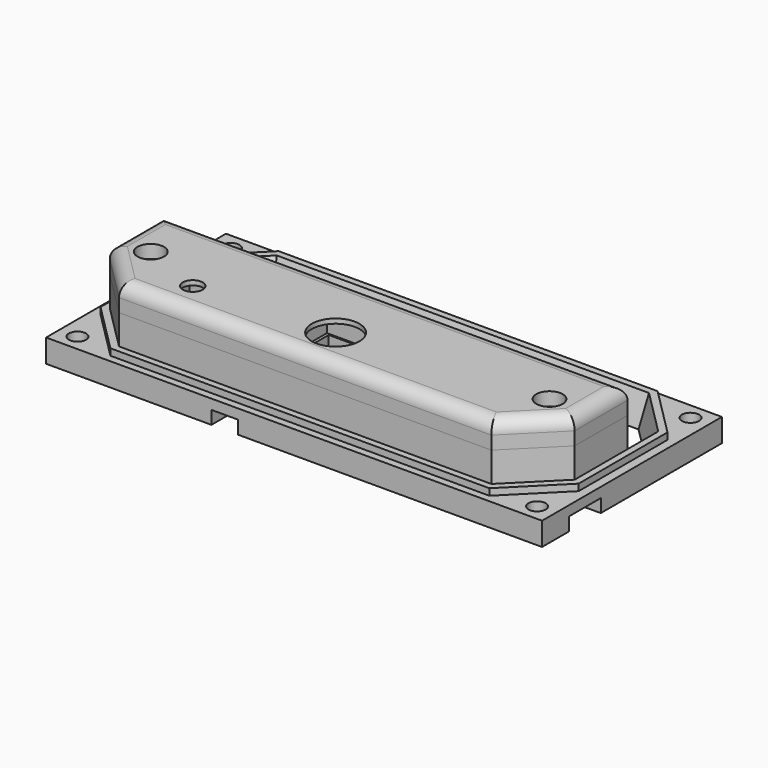
from build123d import *

# Parameters (mm, degrees)
F0_W              = 75
F0_H              = 34
F0_R              = 1.3
F1_DEPTH          = 3.5
F3_DEPTH          = 1
F5_DEPTH          = 5
F11_DEPTH         = 9
F12_W             = 15
F12_H             = 10
F13_DEPTH         = 8.5
F14_W             = 7.3
F14_H             = 4.5
F15_DEPTH         = 5
F16_W             = 9
F16_H             = 10
F16_W_2           = 7
F16_H_2           = 4
F17_DEPTH         = 25
F18_W             = 2
F18_H             = 5
F19_DEPTH         = 10
F20_W             = 6
F20_H             = 2
F21_DEPTH         = 25
F22_R             = 0.8
F23_DEPTH         = 5
F26_DEPTH         = 4
F27_R             = 3.6
F27_R_2           = 1.5
F28_DEPTH         = 25
F29_W             = 13
F29_H             = 10.5
F29_W_2           = 8
F29_H_2           = 5
F30_DEPTH         = 3.3
F31_W             = 2
F31_H             = 4
F32_DEPTH         = 7
F33_W             = 4
F33_H             = 2
F34_DEPTH         = 25
F36_D             = 2
F36_DEPTH         = 10
F36_CBORE_D       = 4
F36_CBORE_DEPTH   = 2
F36_TIP           = 0.600860619
F36_2_D           = 2
F36_2_DEPTH       = 10
F36_2_CBORE_D     = 4
F36_2_CBORE_DEPTH = 2
F36_2_TIP         = 0.600860619
F37_R             = 2


with BuildPart() as f1:
    # F0 (on Top) → F1 (new body)
    with BuildSketch(Plane.XY):
        Rectangle(F0_W, F0_H)
        with Locations((-34.75, -14.5)):
            Circle(F0_R, mode=Mode.SUBTRACT)
        with Locations((34.75, -14.5)):
            Circle(F0_R, mode=Mode.SUBTRACT)
        with Locations((-34.75, 14.5)):
            Circle(F0_R, mode=Mode.SUBTRACT)
        with Locations((34.75, 14.5)):
            Circle(F0_R, mode=Mode.SUBTRACT)
    extrude(amount=F1_DEPTH)

    # F2 (on face) → F3 (join)
    with BuildSketch(Plane.XY.offset(3.5)):
        Polygon((28.65, 15.9), (-28.65, 15.9), (-36.15, 8.4), (-36.15, -8.4), (-28.65, -15.9), (28.65, -15.9), (36.15, -8.4), (36.15, 8.4), align=None)
    extrude(amount=F3_DEPTH)

    # F4 (on face) → F5 (cut)
    with BuildSketch(Plane.XY.offset(4.5)):
        Polygon((28.15, 14.9), (-28.15, 14.9), (-35.15, 7.9), (-35.15, -7.9), (-28.15, -14.9), (28.15, -14.9), (35.15, -7.9), (35.15, 7.9), align=None)
    extrude(amount=-F5_DEPTH, mode=Mode.SUBTRACT)

    # F9: sweep along a path in F8
    with BuildLine(Plane.XY.offset(4.5)) as f9_path:
        Line((-35.15, 2.1), (-35.15, 7.9))
        Line((-35.15, 7.9), (-28.15, 14.9))
        Line((-28.15, 14.9), (28.15, 14.9))
        Line((28.15, 14.9), (35.15, 7.9))
        Line((35.15, 7.9), (35.15, 2.1))
    # F7 (on offset) → F9 (sweep)
    with BuildSketch(Plane.XZ.offset(-2.1)):
        Polygon((-33.85, 0), (-35.15, 4.5), (-35.15, 0), align=None)
    sweep(path=f9_path.line, transition=Transition.RIGHT)

    # F10 (on Top) → F11 (join)
    with BuildSketch(Plane.XY):
        Polygon((-35.15, -7.9), (-28.15, -14.9), (28.15, -14.9), (35.15, -7.9), (35.15, 2.1), (-35.15, 2.1), align=None)
    extrude(amount=F11_DEPTH)

    # F12 (on face) → F13 (cut)
    with BuildSketch(Plane.XY.offset(9)):
        with Locations((2.25, -8.9)):
            Rectangle(F12_W, F12_H)
    extrude(amount=-F13_DEPTH, mode=Mode.SUBTRACT)

    # F14 (on face) → F15 (cut)
    with BuildSketch(Plane.XY.offset(9)):
        with Locations((-19.15, -10.15)):
            Rectangle(F14_W, F14_H)
    extrude(amount=-F15_DEPTH, mode=Mode.SUBTRACT)

    # F16 (on face) → F17 (cut)
    with BuildSketch(Plane.XY.offset(9)):
        with Locations((14.25, -8.9)):
            Rectangle(F16_W, F16_H)
        with Locations((-12, -10.15)):
            Rectangle(F16_W_2, F16_H_2)
    extrude(amount=-F17_DEPTH, mode=Mode.SUBTRACT)

    # F18 (on face) → F19 (join)
    with BuildSketch(Plane.XZ.offset(3.9)):
        with Locations((15.25, 2.5)):
            Rectangle(F18_W, F18_H)
    extrude(amount=F19_DEPTH)

    # F20 (on face) → F21 (cut)
    with BuildSketch(Plane(origin=(14.25, 0, 0), x_dir=(0, -1, 0), z_dir=(-1, 0, 0))):
        with Locations((8.9, 1)):
            Rectangle(F20_W, F20_H)
    extrude(amount=-F21_DEPTH, mode=Mode.SUBTRACT)

    # F22 (on face) → F23 (cut)
    with BuildSketch(Plane.XY.offset(9)):
        with Locations((-30.15, -6.4)):
            Circle(F22_R)
        with Locations((30.15, -6.4)):
            Circle(F22_R)
    extrude(amount=-F23_DEPTH, mode=Mode.SUBTRACT)

    # F31 (on face) → F32 (join)
    with BuildSketch(Plane.YZ.offset(-15.5)):
        with Locations((-10.15, 2)):
            Rectangle(F31_W, F31_H)
    extrude(amount=F32_DEPTH)

    # F33 (on face) → F34 (cut)
    with BuildSketch(Plane(origin=(0, -9.15, 0), x_dir=(-1, 0, 0), z_dir=(0, 1, 0))):
        with Locations((10.5, 1)):
            Rectangle(F33_W, F33_H)
    extrude(amount=-F34_DEPTH, mode=Mode.SUBTRACT)

    # F36
    with Locations(Plane.XY.offset(13)):
        with Locations((-30.15, -6.4), (30.15, -6.4)):
            CounterBoreHole(F36_D / 2, F36_CBORE_D / 2, F36_CBORE_DEPTH, depth=F36_DEPTH)
            with Locations((0, 0, -(F36_DEPTH + F36_TIP / 2))):  # 118° drill point
                Cone(0, F36_D / 2, F36_TIP, mode=Mode.SUBTRACT)


with BuildPart() as f26:
    # F25 (on offset) → F26 (new body)
    with BuildSketch(Plane.XY.offset(9)):
        Polygon((-35.15, -7.9), (-28.15, -14.9), (28.15, -14.9), (35.15, -7.9), (35.15, 2.1), (-35.15, 2.1), align=None)
    extrude(amount=F26_DEPTH)

    # F27 (on face) → F28 (cut)
    with BuildSketch(Plane.XY.offset(13)):
        with Locations((-0.2, -8.9)):
            Circle(F27_R)
        with Locations((-20.8, -10.15)):
            Circle(F27_R_2)
    extrude(amount=-F28_DEPTH, mode=Mode.SUBTRACT)

    # F29 (on face) → F30 (cut)
    with BuildSketch(Plane(origin=(0, 0, 9), x_dir=(1, 0, 0), z_dir=(0, 0, -1))):
        with Locations((0.8, 8.9)):
            Rectangle(F29_W, F29_H)
        with Locations((-19.3, 10.15)):
            Rectangle(F29_W_2, F29_H_2)
    extrude(amount=-F30_DEPTH, mode=Mode.SUBTRACT)

    # F36#2
    with Locations(Plane.XY.offset(13)):
        with Locations((-30.15, -6.4), (30.15, -6.4)):
            CounterBoreHole(F36_2_D / 2, F36_2_CBORE_D / 2, F36_2_CBORE_DEPTH, depth=F36_2_DEPTH)
            with Locations((0, 0, -(F36_2_DEPTH + F36_2_TIP / 2))):  # 118° drill point
                Cone(0, F36_2_D / 2, F36_2_TIP, mode=Mode.SUBTRACT)

    # F37
    f37_edges = [f26.edges().sort_by_distance(p)[0] for p in [
        (0, -14.9, 13),
        (-31.65, -11.4, 13),
        (-35.15, -2.9, 13),
        (0, 2.1, 13),
        (35.15, -2.9, 13),
        (31.65, -11.4, 13),
    ]]
    fillet(f37_edges, radius=F37_R)


solid = Compound([f1.part, f26.part])
